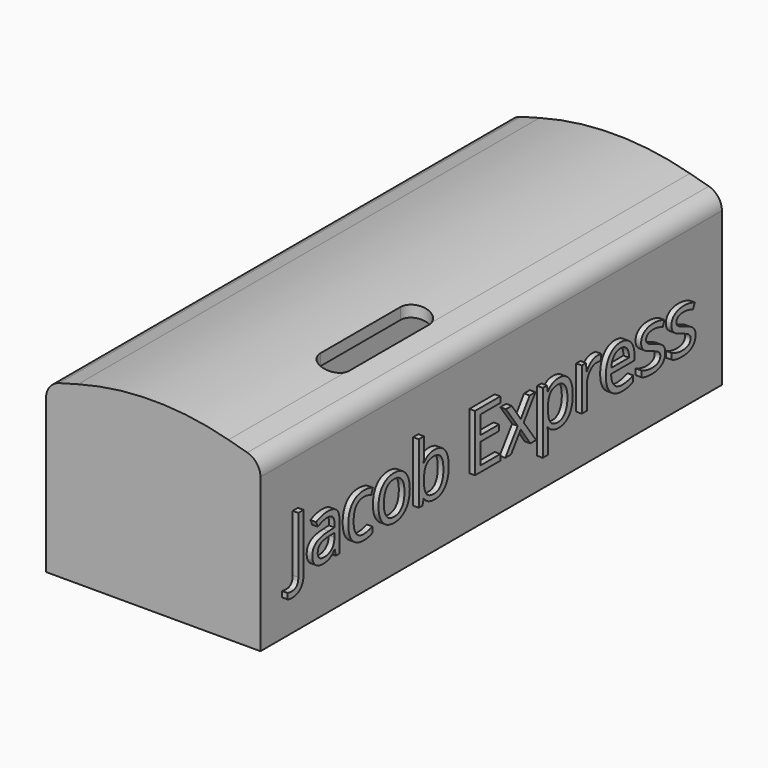
from build123d import *

# Parameters (mm, degrees)
F4_DEPTH      = 44.9707
F4_DEPTH_BACK = 57.5437
F5_T          = -2
F6_DEPTH      = 33.021
F7_R          = 11.1125
F8_DEPTH      = 2
F9_TEXT_SIZE  = 14.1111111111
F10_DEPTH     = 1
F11_TEXT_SIZE = 14.1111111111
F12_DEPTH     = 1


# Not quite as in the source:
# - Text() gives the source's letters only with a copy of the font that has no kerning and outlines rounded to 1/6400 em; it was checked with that copy


with BuildPart() as f4:
    # F3 (on Front) → F4 (new body, two sides)
    with BuildSketch(Plane.XZ) as f4_sk:
        with BuildLine():
            Line((-19.05, 27.2550562345), (-19.05, 0))
            Line((-19.05, 0), (19.05, 0))
            Line((19.05, 0), (19.05, 27.2550562345))
            ThreePointArc((19.05, 27.2550562345), (18.3981431874, 29.1823272211), (16.7102371932, 30.3182251542))
            Line((16.7102371932, 30.3182251542), (13.3637950915, 31.2307027164))
            ThreePointArc((13.3637950915, 31.2307027164), (0, 33.02), (-13.3637950915, 31.2307027164))
            Line((-13.3637950915, 31.2307027164), (-16.7102371932, 30.3182251542))
            ThreePointArc((-16.7102371932, 30.3182251542), (-18.3981431874, 29.1823272211), (-19.05, 27.2550562345))
        make_face()
    extrude(amount=F4_DEPTH)
    extrude(f4_sk.sketch, amount=-F4_DEPTH_BACK)

    # F5
    f5_openings = [f4.faces().sort_by_distance(p)[0] for p in [
        (0, 6.2865, 0),
    ]]
    offset(amount=F5_T, openings=f5_openings)

    # F2 (on Top) → F6 (cut, through all)
    with BuildSketch(Plane.XY):
        with BuildLine():
            Line((13.462, -18.3007), (13.462, -0.5207))
            ThreePointArc((13.462, -0.5207), (10.922, 2.0193), (8.382, -0.5207))
            Line((8.382, -0.5207), (8.382, -18.3007))
            ThreePointArc((8.382, -18.3007), (10.922, -20.8407), (13.462, -18.3007))
        make_face()
    extrude(amount=F6_DEPTH, mode=Mode.SUBTRACT)

    # F7 (on face) → F8 (join)
    with BuildSketch(Plane(origin=(0, 57.5437, 0), x_dir=(-1, 0, 0), z_dir=(0, 1, 0))):
        with Locations((0, 17.0895773917)):
            Circle(F7_R)
    extrude(amount=F8_DEPTH)

    # F9 (on face) → F10 (join)
    with BuildSketch(Plane(origin=(-19.05, 0, 0), x_dir=(0, -1, 0), z_dir=(-1, 0, 0))):
        with Locations((-51.8835627701, 9.0687419797)):
            Text('Jacob Express', F9_TEXT_SIZE, font='Open Sans', text_align=(TextAlign.LEFT, TextAlign.BOTTOM))
    extrude(amount=F10_DEPTH)

    # F11 (on face) → F12 (join)
    with BuildSketch(Plane.YZ.offset(19.05)):
        with Locations((-39.1167592177, 8.9801382525)):
            Text('Jacob Express', F11_TEXT_SIZE, font='Open Sans', text_align=(TextAlign.LEFT, TextAlign.BOTTOM))
    extrude(amount=F12_DEPTH)


solid = f4.part
